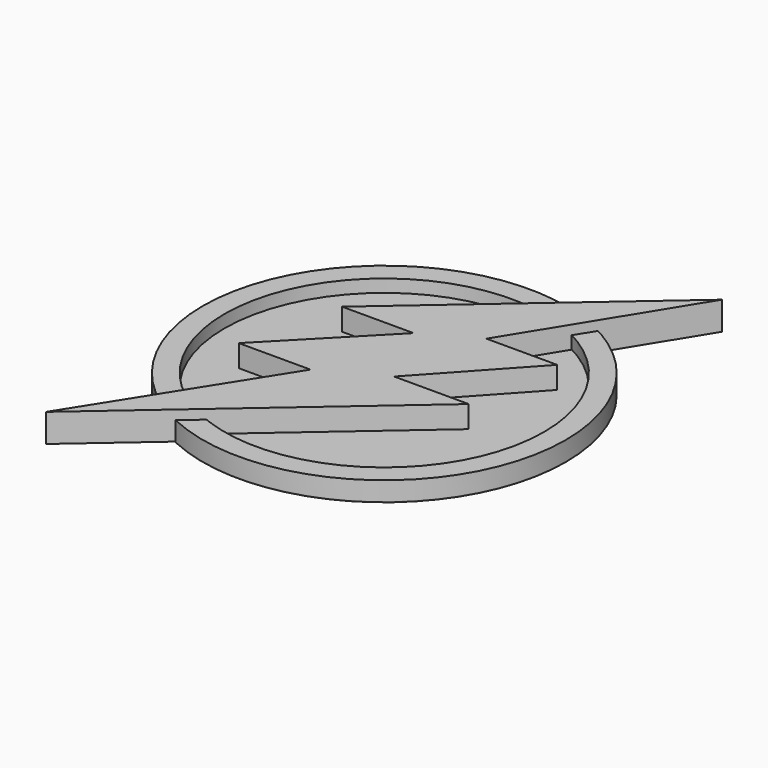
from build123d import *

# Parameters (mm, degrees)
F1_R     = 29.346135088
F1_R_2   = 25.8393981861
F5_DEPTH = 1
F6_DEPTH = 0.1
F7_DEPTH = 3.048
F8_DEPTH = 4.572


# Not quite as in the source:
# - the program builds the solid bodies; features that only make, move or delete a surface that nothing else refers to are left out


with BuildPart() as f5:
    # F1 (on face) → F5 (new body)
    with BuildSketch(Plane.XY):
        Circle(F1_R)
        Circle(F1_R_2, mode=Mode.SUBTRACT)
        Circle(F1_R_2)
    extrude(amount=F5_DEPTH)


with BuildPart() as f6:
    # F1 (on face) → F6 (new body)
    with BuildSketch(Plane.XY):
        Circle(F1_R)
        Circle(F1_R_2, mode=Mode.SUBTRACT)
        Circle(F1_R_2)
    extrude(amount=-F6_DEPTH)


with BuildPart() as f7:
    # F1 (on face) → F7 (new body)
    with BuildSketch(Plane.XY):
        Circle(F1_R)
        Circle(F1_R_2, mode=Mode.SUBTRACT)
    extrude(amount=F7_DEPTH)


with BuildPart() as f8:
    # F2 (on Top) → F8 (new body)
    with BuildSketch(Plane.XY):
        Polygon((6.0379398285, 13.0822043866), (22.5992734988, 39.9943725895), (-13.6509970043, 8.5318721831), (-2.0855690818, 8.5318721831), (-17.6184918681, -7.3942895979), (-6.025892119, -7.3942895979), (-24.8665944569, -37.2795380606), (15.4645281288, -2.2751658689), (3.412750084, -2.2751658689), (17.4903385899, 13.0822043866), align=None)
    extrude(amount=F8_DEPTH)


solid = Compound([f5.part, f6.part, f7.part, f8.part])
